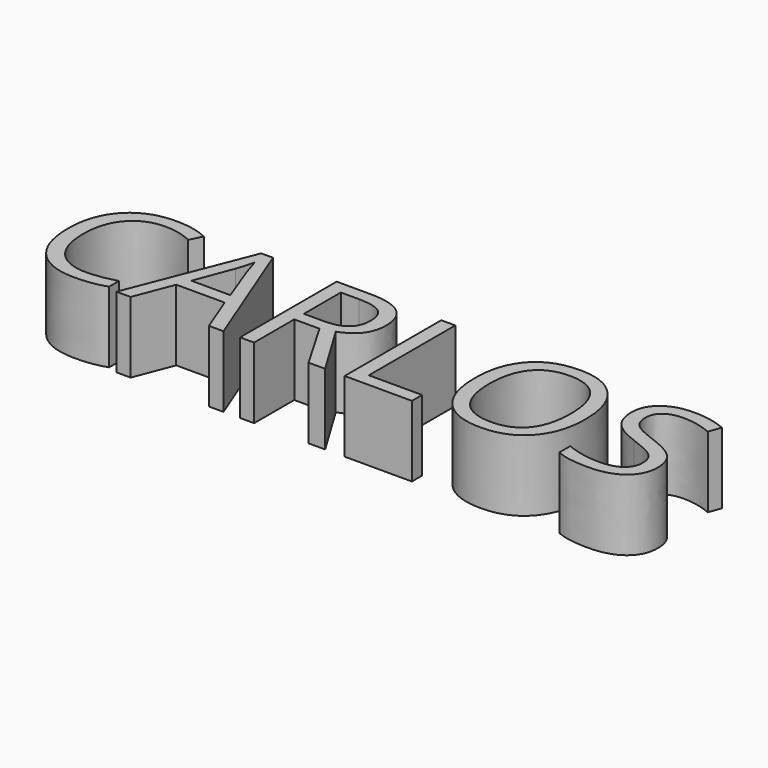
from build123d import *

# Parameters (mm, degrees)
F0_TEXT_SIZE = 59.5414215544
F1_DEPTH     = 25


# Not quite as in the source:
# - Text() gives the source's letters only with a copy of the font that has no kerning and outlines rounded to 1/6400 em; it was checked with that copy


with BuildPart() as f1:
    # F0 (on Top) → F1 (new body)
    with BuildSketch(Plane.XY):
        with Locations((-57.3150925338, 4.0384619497)):
            Text('CARLOS', F0_TEXT_SIZE, font='Open Sans', text_align=(TextAlign.LEFT, TextAlign.BOTTOM))
    extrude(amount=F1_DEPTH)


solid = f1.part
